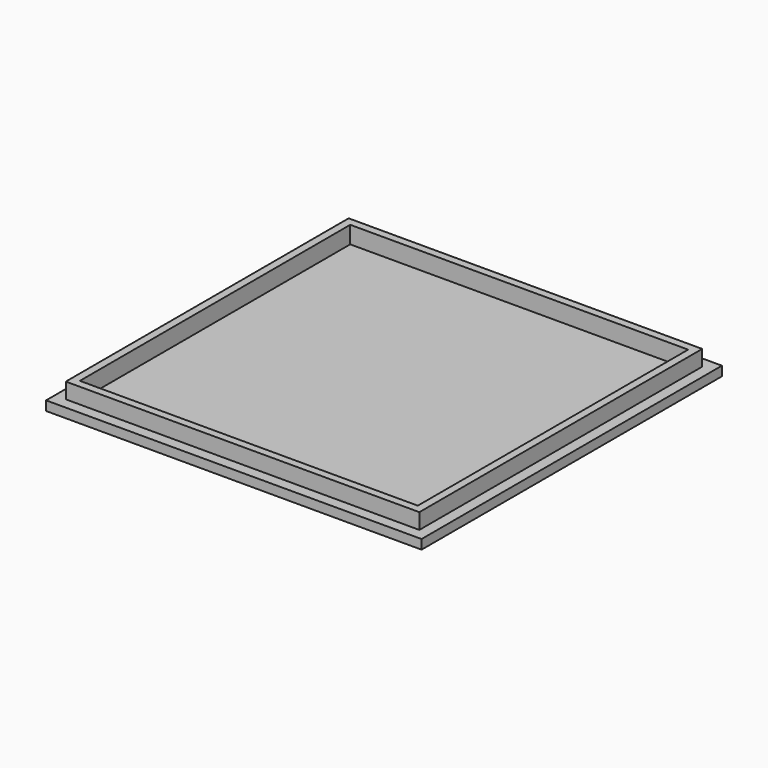
from build123d import *

# Parameters (mm, degrees)
F0_W        = 120
F0_H        = 120
F1_DEPTH    = 3
F2_W        = 113
F2_H        = 113
F3_DEPTH    = 5
F4_T        = 2.5
F4_T3_DEPTH = 118
F4_T5_DEPTH = 118


# Not quite as in the source:
# - a shell that OpenCascade refuses in one call is made with other operations: the cavity is built on its own and cut out


with BuildPart() as f1:
    # F0 (on Top) → F1 (new body)
    with BuildSketch(Plane.XY):
        Rectangle(F0_W, F0_H)
    extrude(amount=F1_DEPTH)

    # F2 (on face) → F3 (join)
    with BuildSketch(Plane.XY.offset(3)):
        Rectangle(F2_W, F2_H)
    extrude(amount=F3_DEPTH)

    # F4: shell of thickness 2.5, made by hand


with BuildPart() as f4_core1:
    # F4_t2: copy of F1
    add(f1.part)

    # the walls: a layer under each face that stays
    f4_faces = [f4_core1.faces().sort_by_distance(p)[0] for p in [
        (0, -60, 1.5),
        (-60, 0, 1.5),
        (60, 0, 1.5),
        (0, 0, 0),
        (41.25, -58.5185185185, 3),
        (0, 60, 1.5),
        (0, -56.5, 5.5),
        (56.5, 0, 5.5),
        (0, 56.5, 5.5),
        (-56.5, 0, 5.5),
    ]]
    thicken(f4_faces, amount=-F4_T, mode=Mode.SUBTRACT)

    # F4_s4 → F4_t3 (cut)
    with BuildSketch(Plane.YZ.offset(-59)):
        Polygon((-56.525, 3.025), (-56.5, 0.5), (-54, 0.5), (-54, 3), align=None)
        Polygon((56.525, 3.025), (56.5, 0.5), (54, 0.5), (54, 3), align=None)
    extrude(amount=F4_T3_DEPTH, mode=Mode.SUBTRACT)

    # F4_s6 → F4_t5 (cut)
    with BuildSketch(Plane.XZ.offset(-59)):
        Polygon((56.525, 3.025), (56.5, 0.5), (54, 0.5), (54, 3), align=None)
        Polygon((-56.525, 3.025), (-56.5, 0.5), (-54, 0.5), (-54, 3), align=None)
    extrude(amount=F4_T5_DEPTH, mode=Mode.SUBTRACT)


with BuildPart() as f1_1:
    add(f1.part)

    # what is left inside the walls is the cavity
    f4_cavity = [f4_core1.part.solids().sort_by_distance(p)[0] for p in [
        (0, -18, 2.525),
    ]]
    add(f4_cavity, mode=Mode.SUBTRACT)


solid = f1_1.part
